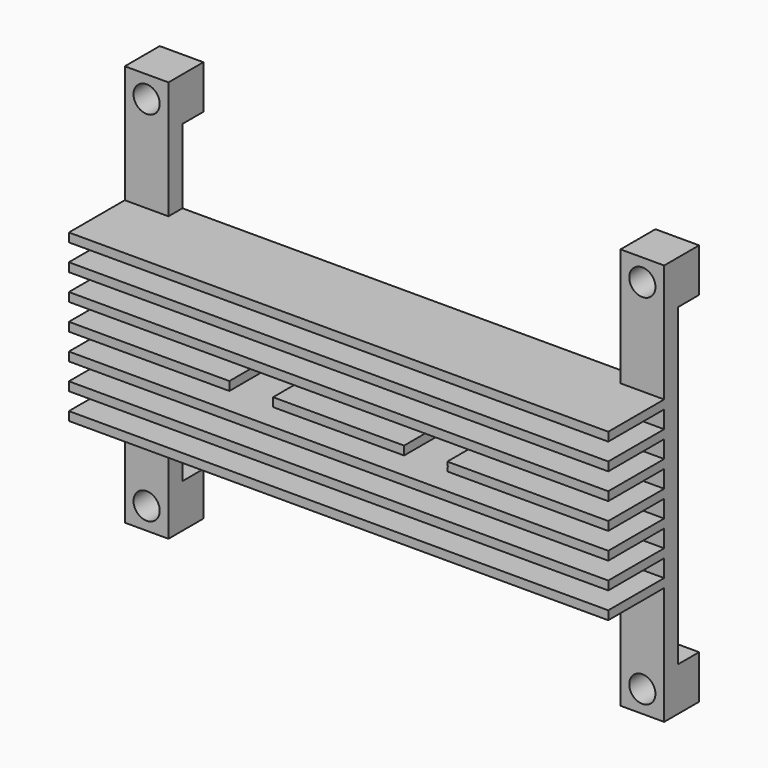
from build123d import *

# Parameters (mm, degrees)
F1_DEPTH = 10
F2_W     = 5
F2_H     = 13.5
F2_W_2   = 61.75
F2_H_2   = 2
F4_DEPTH = 8
F5_W     = 5
F5_H     = 5
F5_R     = 1.5
F5_R_2   = 0.9
F5_W_2   = 4.6
F5_H_2   = 6.1
F7_DEPTH = 5
F8_DEPTH = 8.001
F9_DEPTH = 5.001


# Not quite as in the source:
# - a feature names something its author has since deleted; it is built from what else it names


with BuildPart() as f1:
    # F0 (on Front) → F1 (new body)
    with BuildSketch(Plane.XZ):
        Polygon((-25.875, 23), (-30.875, 23), (-30.875, -23), (-25.875, -23), (-25.875, -9.5), (0, -9.5), (25.875, -9.5), (25.875, -23), (30.875, -23), (30.875, 23), (25.875, 23), (25.875, 9.5), (0, 9.5), (-25.875, 9.5), align=None)
    extrude(amount=F1_DEPTH)

    # F2 (on face) → F4 (cut, through all)
    with BuildSketch(Plane.XZ.offset(10)):
        with Locations((-28.375, 16.25)):
            Rectangle(F2_W, F2_H)
        with Locations((0, 7.5)):
            Rectangle(F2_W_2, F2_H_2)
        with Locations((0, 4.5)):
            Rectangle(F2_W_2, F2_H_2)
        with Locations((0, 1.5)):
            Rectangle(F2_W_2, F2_H_2)
        with Locations((0, -1.5)):
            Rectangle(F2_W_2, F2_H_2)
        with Locations((0, -4.5)):
            Rectangle(F2_W_2, F2_H_2)
        with Locations((0, -7.5)):
            Rectangle(F2_W_2, F2_H_2)
        with Locations((-28.375, -16.25)):
            Rectangle(F2_W, F2_H)
        with Locations((28.375, 16.25)):
            Rectangle(F2_W, F2_H)
        with Locations((28.375, -16.25)):
            Rectangle(F2_W, F2_H)
    extrude(amount=-F4_DEPTH, mode=Mode.SUBTRACT)

    # F5 (on offset) → F7 (join, through all)
    with BuildSketch(Plane.XZ.offset(2)):
        with Locations((-28.375, 20.5)):
            Rectangle(F5_W, F5_H)
        with Locations((-28.375, 20.5)):
            Circle(F5_R, mode=Mode.SUBTRACT)
        with Locations((28.375, 20.5)):
            Rectangle(F5_W, F5_H)
        with Locations((28.375, 20.5)):
            Circle(F5_R, mode=Mode.SUBTRACT)
        with Locations((28.375, -20.5)):
            Rectangle(F5_W, F5_H)
        with Locations((28.375, -20.5)):
            Circle(F5_R, mode=Mode.SUBTRACT)
        with Locations((-28.375, -20.5)):
            Rectangle(F5_W, F5_H)
        with Locations((-28.375, -20.5)):
            Circle(F5_R, mode=Mode.SUBTRACT)
        with BuildLine():
            ThreePointArc((10, 2.5), (8.232233047, 1.767766953), (7.5, 0))
            ThreePointArc((7.5, 0), (8.232233047, -1.767766953), (10, -2.5))
            ThreePointArc((10, -2.5), (11.767766953, -1.767766953), (12.5, 0))
            ThreePointArc((12.5, 0), (11.767766953, 1.767766953), (10, 2.5))
        make_face()
        with Locations((10, 0)):
            Circle(F5_R_2, mode=Mode.SUBTRACT)
        with BuildLine():
            ThreePointArc((-10, -2.5), (-8.232233047, -1.767766953), (-7.5, 0))
            ThreePointArc((-7.5, 0), (-8.232233047, 1.767766953), (-10, 2.5))
            ThreePointArc((-10, 2.5), (-11.767766953, 1.767766953), (-12.5, 0))
            ThreePointArc((-12.5, 0), (-11.767766953, -1.767766953), (-10, -2.5))
        make_face()
        with Locations((-10, 0)):
            Circle(F5_R_2, mode=Mode.SUBTRACT)
        with Locations((0, -1.25)):
            Rectangle(F5_W_2, F5_H_2)
    extrude(amount=-F7_DEPTH)

    # F5 (on offset) → F8 (cut, through all)
    with BuildSketch(Plane.XZ.offset(2)):
        with BuildLine():
            ThreePointArc((-10, 2.5), (-8.232233047, 1.767766953), (-7.5, 0))
            Line((-7.5, 0), (-7.5, 2.5))
            Line((-7.5, 2.5), (-10, 2.5))
        make_face()
        with BuildLine():
            ThreePointArc((-12.5, 0), (-11.767766953, 1.767766953), (-10, 2.5))
            Line((-10, 2.5), (-12.5, 2.5))
            Line((-12.5, 2.5), (-12.5, 0))
        make_face()
        with BuildLine():
            Line((-12.5, -2.5), (-10, -2.5))
            ThreePointArc((-10, -2.5), (-11.767766953, -1.767766953), (-12.5, 0))
            Line((-12.5, 0), (-12.5, -2.5))
        make_face()
        with BuildLine():
            Line((-7.5, -2.5), (-7.5, 0))
            ThreePointArc((-7.5, 0), (-8.232233047, -1.767766953), (-10, -2.5))
            Line((-10, -2.5), (-7.5, -2.5))
        make_face()
        with BuildLine():
            ThreePointArc((-10, -2.5), (-8.232233047, -1.767766953), (-7.5, 0))
            ThreePointArc((-7.5, 0), (-8.232233047, 1.767766953), (-10, 2.5))
            ThreePointArc((-10, 2.5), (-11.767766953, 1.767766953), (-12.5, 0))
            ThreePointArc((-12.5, 0), (-11.767766953, -1.767766953), (-10, -2.5))
        make_face()
        with Locations((-10, 0)):
            Circle(F5_R_2, mode=Mode.SUBTRACT)
        with Locations((-10, 0)):
            Circle(F5_R_2)
        with BuildLine():
            Line((10, 2.5), (7.5, 2.5))
            Line((7.5, 2.5), (7.5, 0))
            ThreePointArc((7.5, 0), (8.232233047, 1.767766953), (10, 2.5))
        make_face()
        with BuildLine():
            ThreePointArc((10, -2.5), (8.232233047, -1.767766953), (7.5, 0))
            Line((7.5, 0), (7.5, -2.5))
            Line((7.5, -2.5), (10, -2.5))
        make_face()
        with BuildLine():
            ThreePointArc((10, 2.5), (8.232233047, 1.767766953), (7.5, 0))
            ThreePointArc((7.5, 0), (8.232233047, -1.767766953), (10, -2.5))
            ThreePointArc((10, -2.5), (11.767766953, -1.767766953), (12.5, 0))
            ThreePointArc((12.5, 0), (11.767766953, 1.767766953), (10, 2.5))
        make_face()
        with Locations((10, 0)):
            Circle(F5_R_2, mode=Mode.SUBTRACT)
        with Locations((10, 0)):
            Circle(F5_R_2)
    extrude(amount=F8_DEPTH, mode=Mode.SUBTRACT)

    # F5 (on offset) → F9 (cut, through all)
    with BuildSketch(Plane.XZ.offset(2)):
        with Locations((28.375, 20.5)):
            Circle(F5_R)
        with Locations((10, 0)):
            Circle(F5_R_2)
        with Locations((-10, 0)):
            Circle(F5_R_2)
        with Locations((28.375, -20.5)):
            Circle(F5_R)
        with Locations((-28.375, -20.5)):
            Circle(F5_R)
        with Locations((-28.375, 20.5)):
            Circle(F5_R)
    extrude(amount=-F9_DEPTH, mode=Mode.SUBTRACT)


solid = f1.part
